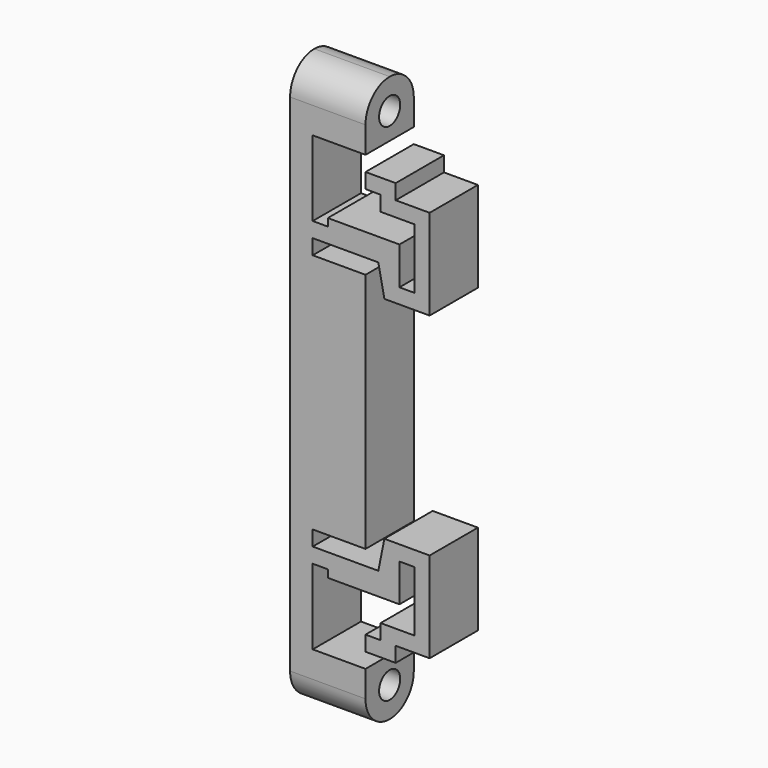
from build123d import *

# Parameters (mm, degrees)
F1_DEPTH    = 8
F2_T4_DEPTH = 33.981320863
F3_T4_DEPTH = 33.981320863
F4_R        = 3.99999
F5_R        = 1.75
F6_DEPTH    = 10
F7_R        = 1.75
F8_DEPTH    = 10


# Not quite as in the source:
# - a fillet or chamfer that OpenCascade refuses, or shapes differently, is made with other operations: its cross-section is extruded or revolved along the edge and cut away or added
# - a fillet or chamfer is up to 0.001 mm smaller than in the source, because OpenCascade refuses the exact size


with BuildPart() as f1:
    # F0 (on Front) → F1 (new body)
    with BuildSketch(Plane.XZ):
        Polygon((14, 65.5), (10, 65.5), (10, 63.5), (12, 63.5), (12, 61.5), (16.5, 61.5), (16.5, 58.5), (16.5, 53.5), (14.5, 53.5), (14.5, 58.5), (10, 58.5), (10, 55.5), (11.5, 55.5), (11.5, 51.5), (18.5, 51.5), (18.5, 63.5), (14, 63.5), align=None)
        Polygon((10, 11.5), (10, 9.5), (14, 9.5), (14, 11.5), (18.5, 11.5), (18.5, 23.5), (11.5, 23.5), (11.5, 19.5), (10, 19.5), (10, 16.5), (14.5, 16.5), (14.5, 21.5), (16.5, 21.5), (16.5, 16.5), (16.5, 13.5), (12, 13.5), (12, 11.5), align=None)
        Polygon((0, 75), (0, 0), (10, 0), (10, 7.5), (3, 7.5), (3, 9.5), (3, 13.5), (3, 16.5), (3, 17.5), (5, 17.5), (5, 16.5), (10, 16.5), (10, 19.5), (3, 19.5), (3, 21.5), (10, 21.5), (10, 53.5), (3, 53.5), (3, 55.5), (10, 55.5), (10, 58.5), (5, 58.5), (5, 57.5), (3, 57.5), (3, 58.5), (3, 61.5), (3, 65.5), (3, 67.5), (10, 67.5), (10, 75), align=None)
    extrude(amount=F1_DEPTH)

    # F2: chamfer of 1 x 5 on 1 edges, made by hand


with BuildPart() as f2_tool2:
    # F2_s3 → F2_t4 (new body)
    with BuildSketch(Plane.XZ.offset(-12.9906604315)):
        Polygon((11.5, 56.5), (12.5, 51.5), (11.5, 51.5), align=None)
    extrude(amount=F2_T4_DEPTH)

    split(bisect_by=Plane.XY.offset(55.5), keep=Keep.BOTTOM)


with BuildPart() as f1_1:
    add(f1.part)

    # F2_t1: cut F2_tool2
    add(f2_tool2.part, mode=Mode.SUBTRACT)

    # F3: chamfer of 5 x 1 on 1 edges, made by hand


with BuildPart() as f3_tool2:
    # F3_s3 → F3_t4 (new body)
    with BuildSketch(Plane.XZ.offset(-12.9906604315)):
        Polygon((11.5, 18.5), (12.5, 23.5), (11.5, 23.5), align=None)
    extrude(amount=F3_T4_DEPTH)

    split(bisect_by=Plane.XY.offset(19.5), keep=Keep.TOP)


with BuildPart() as f1_2:
    add(f1_1.part)

    # F3_t1: cut F3_tool2
    add(f3_tool2.part, mode=Mode.SUBTRACT)

    # F4 (radius 4 in the source; OpenCascade refuses exactly that, so slightly less here)
    f4_edges = [f1_2.edges().sort_by_distance(p)[0] for p in [
        (5, -8, 75),
        (5, 0, 75),
        (5, -8, 0),
        (5, 0, 0),
    ]]
    fillet(f4_edges, radius=F4_R)

    # F5 (on face) → F6 (cut)
    with BuildSketch(Plane.YZ.offset(10)):
        with Locations((-4, 71)):
            Circle(F5_R)
    extrude(amount=-F6_DEPTH, mode=Mode.SUBTRACT)

    # F7 (on face) → F8 (cut)
    with BuildSketch(Plane.YZ.offset(10)):
        with Locations((-4, 4)):
            Circle(F7_R)
    extrude(amount=-F8_DEPTH, mode=Mode.SUBTRACT)


solid = f1_2.part
